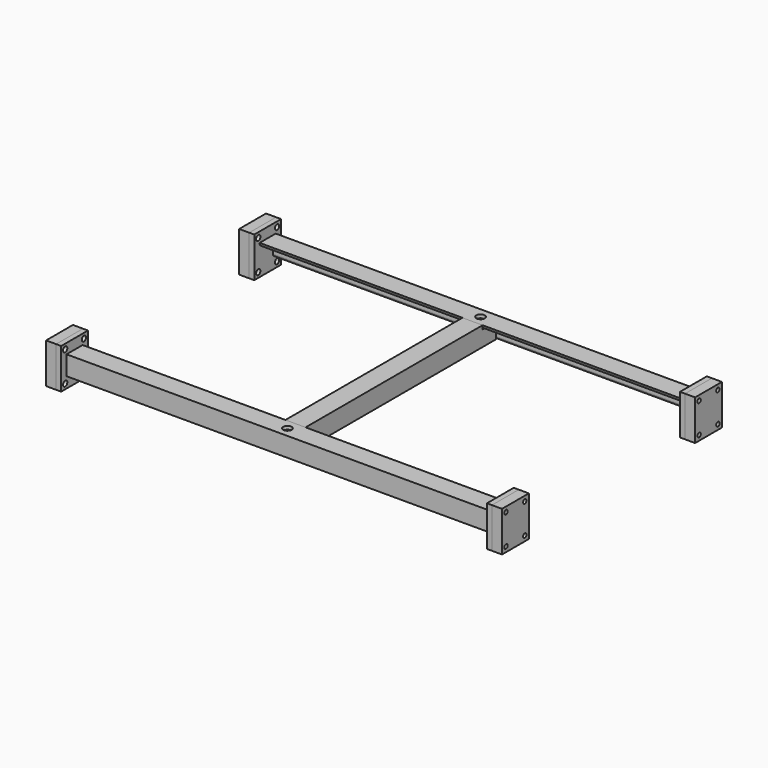
from build123d import *

# Parameters (mm, degrees)
F0_W      = 63.5
F0_H      = 76.2
F1_DEPTH  = 19.05
F4_D      = 7.9375
F8_W      = 63.5
F8_H      = 76.2
F9_DEPTH  = 9.525
F11_D     = 10.0838
F15_DEPTH = 806.45
F19_DEPTH = 482.6
F20_W     = 38.1
F20_H     = 31.75
F21_DEPTH = 7.112
F23_D     = 15.875
F23_2_D   = 15.875


# Not quite as in the source:
# - a length typed as a fraction of an inch, garbled in the dataset ("3 / 203.2 mm" for 3/8 in), is restored


with BuildPart() as f1:
    # F0 (on Right) → F1 (new body)
    with BuildSketch(Plane.YZ):
        Rectangle(F0_W, F0_H)
    extrude(amount=F1_DEPTH)

    # F4 (through all)
    with Locations(Plane.YZ.offset(19.05)):
        with Locations((-22.225, 28.575), (22.225, 28.575), (-22.225, -28.575), (22.225, -28.575)):
            Hole(F4_D / 2)


with BuildPart() as f5_1:
    # F5: instance of F1
    add(f1.part.mirror(Plane(origin=(431.8, 0, 0), x_dir=(0, 1, 0), z_dir=(-1, 0, 0))))


with BuildPart() as f7_1:
    # F7: instance of F1
    add(f1.part.mirror(Plane.XZ.offset(228.6)))


with BuildPart() as f7_2:
    # F7: instance of F5_1
    add(f5_1.part.mirror(Plane.XZ.offset(228.6)))


with BuildPart() as f9:
    # F8 (on face) → F9 (new body)
    with BuildSketch(Plane.YZ.offset(19.05)):
        Rectangle(F8_W, F8_H)
    extrude(amount=F9_DEPTH)

    # F11 (through all)
    with Locations(Plane.YZ.offset(28.575)):
        with Locations((22.225, 28.575), (-22.225, 28.575), (22.225, -28.575), (-22.225, -28.575)):
            Hole(F11_D / 2)


with BuildPart() as f12_1:
    # F12: instance of F9
    add(f9.part.mirror(Plane(origin=(431.8, 0, 0), x_dir=(0, 1, 0), z_dir=(-1, 0, 0))))


with BuildPart() as f13_1:
    # F13: instance of F9
    add(f9.part.mirror(Plane.XZ.offset(228.6)))


with BuildPart() as f13_2:
    # F13: instance of F12_1
    add(f12_1.part.mirror(Plane.XZ.offset(228.6)))


with BuildPart() as f15:
    # F14 (on face) → F15 (new body)
    with BuildSketch(Plane.YZ.offset(28.575)):
        with BuildLine():
            Line((-438.15, 19.05), (-476.25, 19.05))
            Line((-476.25, 19.05), (-476.25, -17.4625))
            Line((-476.25, -17.4625), (-474.6625, -17.4625))
            ThreePointArc((-474.6625, -17.4625), (-471.2949039546, -16.0675960454), (-469.9, -12.7))
            Line((-469.9, -12.7), (-469.9, 6.35))
            ThreePointArc((-469.9, 6.35), (-468.0401280605, 10.8401280605), (-463.55, 12.7))
            Line((-463.55, 12.7), (-442.9125, 12.7))
            ThreePointArc((-442.9125, 12.7), (-439.5449039546, 14.0949039546), (-438.15, 17.4625))
            Line((-438.15, 17.4625), (-438.15, 19.05))
        make_face()
    extrude(amount=F15_DEPTH)


with BuildPart() as f16_1:
    # F16: instance of F15
    add(f15.part.mirror(Plane.XZ.offset(228.6)))

    # F23#2 (through all)
    with Locations(Plane.XY.offset(19.05)):
        with Locations((431.8, -457.2), (431.8, 0)):
            Hole(F23_2_D / 2)


with BuildPart() as f19:
    # F18 (on offset) → F19 (new body)
    with BuildSketch(Plane.XZ.offset(469.9)):
        with BuildLine():
            Line((449.58, -17.4625), (450.85, -17.4625))
            Line((450.85, -17.4625), (450.85, 19.05))
            Line((450.85, 19.05), (412.75, 19.05))
            Line((412.75, 19.05), (412.75, 17.78))
            ThreePointArc((412.75, 17.78), (414.2378975516, 14.1878975516), (417.83, 12.7))
            Line((417.83, 12.7), (438.15, 12.7))
            ThreePointArc((438.15, 12.7), (442.6401280605, 10.8401280605), (444.5, 6.35))
            Line((444.5, 6.35), (444.5, -12.3825))
            ThreePointArc((444.5, -12.3825), (445.9878975516, -15.9746024484), (449.58, -17.4625))
        make_face()
    extrude(amount=-F19_DEPTH)

    # F20 (on face) → F21 (cut)
    with BuildSketch(Plane.XY.offset(19.05)):
        with Locations((431.8, -454.025)):
            Rectangle(F20_W, F20_H)
        with Locations((431.8, -3.175)):
            Rectangle(F20_W, F20_H)
    extrude(amount=-F21_DEPTH, mode=Mode.SUBTRACT)


with BuildPart() as f15_1:
    add(f15.part)

    # F23 (through all)
    with Locations(Plane.XY.offset(19.05)):
        with Locations((431.8, -457.2), (431.8, 0)):
            Hole(F23_D / 2)


solid = Compound([f1.part, f5_1.part, f7_1.part, f7_2.part, f9.part, f12_1.part, f13_1.part, f13_2.part, f16_1.part, f19.part, f15_1.part])
